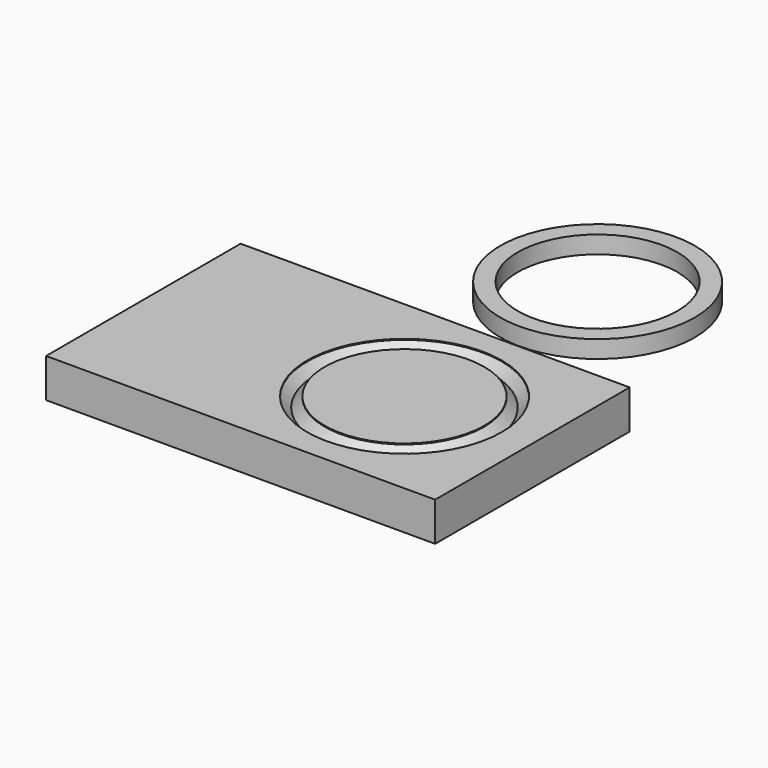
from build123d import *

# Parameters (mm, degrees)
F0_W     = 80
F0_H     = 50
F1_DEPTH = 8
F2_R     = 20
F2_R_2   = 16.4
F3_DEPTH = 3.6
F4_R     = 20
F4_R_2   = 16.4
F5_DEPTH = 2
F6_SIZE  = 1.79999


# Not quite as in the source:
# - a fillet or chamfer is up to 0.001 mm smaller than in the source, because OpenCascade refuses the exact size


with BuildPart() as f1:
    # F0 (on Top) → F1 (new body)
    with BuildSketch(Plane.XY):
        Rectangle(F0_W, F0_H)
    extrude(amount=F1_DEPTH)

    # F4 (on face) → F5 (cut)
    with BuildSketch(Plane.XY.offset(8)):
        with Locations((13.69535923, 0)):
            Circle(F4_R)
        with Locations((13.69535923, 0)):
            Circle(F4_R_2, mode=Mode.SUBTRACT)
    extrude(amount=-F5_DEPTH, mode=Mode.SUBTRACT)

    # F6 (size 1.8 in the source; OpenCascade refuses exactly that, so slightly less here)
    f6_edges = [f1.edges().sort_by_distance(p)[0] for p in [
        (-6.304641, 0, 6),
        (-2.704641, 0, 6),
    ]]
    chamfer(f6_edges, length=F6_SIZE)


with BuildPart() as f3:
    # F2 (on Top) → F3 (new body)
    with BuildSketch(Plane.XY):
        with Locations((7.7231763862, 57.0987015963)):
            Circle(F2_R)
        with Locations((7.7231763862, 57.0987015963)):
            Circle(F2_R_2, mode=Mode.SUBTRACT)
    extrude(amount=F3_DEPTH)


solid = Compound([f1.part, f3.part])
